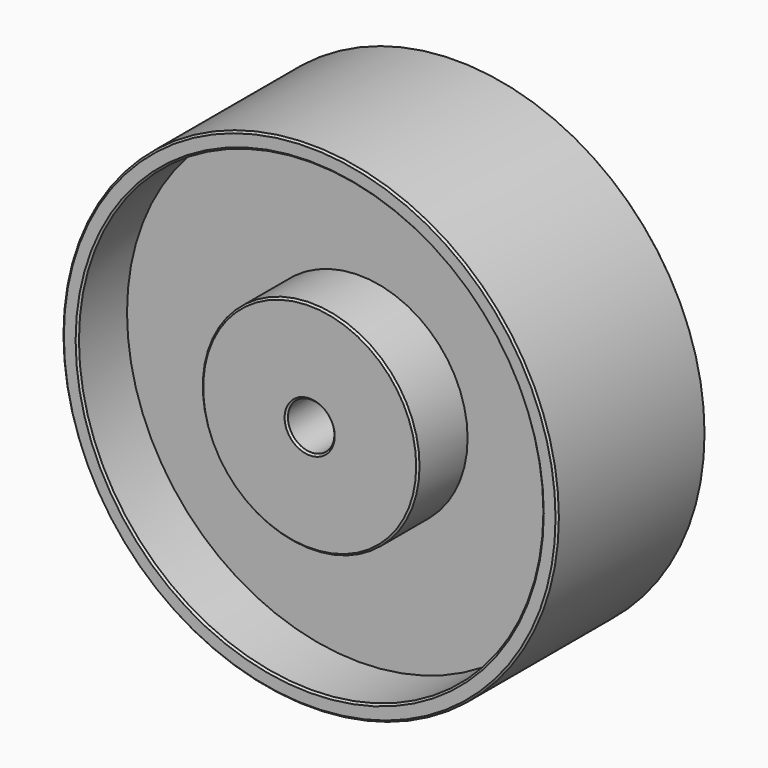
from build123d import *

# Parameters (mm, degrees)
F0_R     = 101.6
F1_DEPTH = 38.1
F2_R     = 95.25
F2_R_2   = 44.45
F3_DEPTH = 25.4
F4_R     = 95.25
F4_R_2   = 44.45
F5_DEPTH = 25.4
F7_D     = 19.05
F8_SIZE  = 0.762


with BuildPart() as f1:
    # F0 (on Front) → F1 (new body, symmetric)
    with BuildSketch(Plane.XZ):
        Circle(F0_R)
    extrude(amount=F1_DEPTH, both=True)

    # F2 (on face) → F3 (cut)
    with BuildSketch(Plane.XZ.offset(38.1)):
        Circle(F2_R)
        Circle(F2_R_2, mode=Mode.SUBTRACT)
    extrude(amount=-F3_DEPTH, mode=Mode.SUBTRACT)

    # F4 (on face) → F5 (cut)
    with BuildSketch(Plane(origin=(0, 38.1, 0), x_dir=(-1, 0, 0), z_dir=(0, 1, 0))):
        Circle(F4_R)
        Circle(F4_R_2, mode=Mode.SUBTRACT)
    extrude(amount=-F5_DEPTH, mode=Mode.SUBTRACT)

    # F7 (through all)
    with Locations(Plane.XZ.offset(38.1)):
        with Locations((0, 0)):
            Hole(F7_D / 2)

    # F8
    f8_edges = [f1.edges().sort_by_distance(p)[0] for p in [
        (-44.45, -38.1, 0),
        (-95.25, -38.1, 0),
        (-101.6, -38.1, 0),
        (44.45, 38.1, 0),
        (95.25, 38.1, 0),
        (-101.6, 38.1, 0),
        (-9.525, 38.1, 0),
        (-9.525, -38.1, 0),
    ]]
    chamfer(f8_edges, length=F8_SIZE)


solid = f1.part
